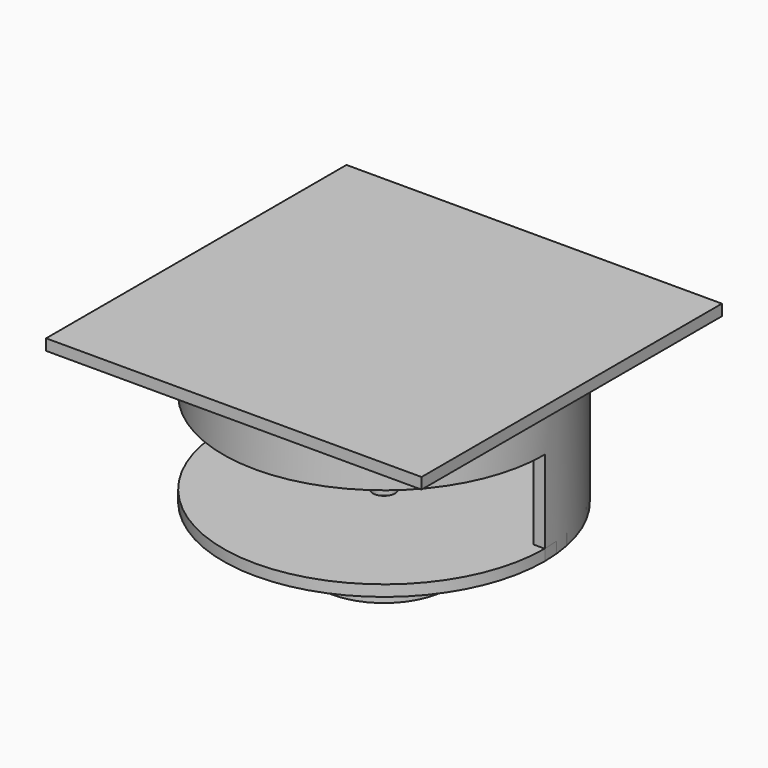
from build123d import *
from build123d import SkipClean  # not in build123d's __all__

# Parameters (mm, degrees)
F1_DEPTH  = 25.4
F2_DEPTH  = 3
F3_R      = 43.5
F3_R_2    = 40.5
F4_DEPTH  = 2
F5_R      = 43.5
F5_R_2    = 40.5
F6_DEPTH  = 12.7
F7_W      = 101.6
F7_H      = 101.6
F8_DEPTH  = 3
F9_R      = 17.5
F9_R_2    = 14
F10_DEPTH = 15
F11_D     = 6
F11_DEPTH = 20
F11_TIP   = 1.8025818571
F12_DEPTH = 3


# Not quite as in the source:
# - after a boolean that leaves OpenCascade's solid faulty, fix() repairs it
# - a feature names something its author has since deleted; it is built from what else it names


with BuildPart() as f1:
    # F0 (on Top) → F1 (new body)
    with BuildSketch(Plane.XY):
        with BuildLine():
            Line((0, 40.5), (0, 43.5))
            ThreePointArc((0, 43.5), (-30.7591449816, 30.7591449816), (-43.5, 0))
            Line((-43.5, 0), (-40.5, 0))
            ThreePointArc((-40.5, 0), (-28.6378246381, 28.6378246381), (0, 40.5))
        make_face()
        with BuildLine():
            Line((40.5, 0), (43.5, 0))
            ThreePointArc((43.5, 0), (30.7591449816, 30.7591449816), (0, 43.5))
            Line((0, 43.5), (0, 40.5))
            ThreePointArc((0, 40.5), (28.6378246381, 28.6378246381), (40.5, 0))
        make_face()
    extrude(amount=F1_DEPTH)

    # F3 (on face) → F4 (join)
    with BuildSketch(Plane.XY.offset(25.4)):
        Circle(F3_R)
        Circle(F3_R_2, mode=Mode.SUBTRACT)
    with SkipClean():  # cleaning this boolean's faces spoils the solid; the shape is the same uncleaned
        extrude(amount=F4_DEPTH)

    # F5 (on face) → F6 (join)
    with BuildSketch(Plane.XY.offset(27.4)):
        Circle(F5_R)
        Circle(F5_R_2, mode=Mode.SUBTRACT)
    extrude(amount=F6_DEPTH)

    add(f1.part.fix(), mode=Mode.REPLACE)

    # F7 (on face) → F8 (join)
    with BuildSketch(Plane.XY.offset(40.1)):
        Rectangle(F7_W, F7_H)
    extrude(amount=F8_DEPTH)


with BuildPart() as f2:
    # F0 (on Top) → F2 (new body)
    with BuildSketch(Plane.XY):
        with BuildLine():
            ThreePointArc((-43.5, 0), (0, -43.5), (43.5, 0))
            Line((43.5, 0), (40.5, 0))
            ThreePointArc((40.5, 0), (28.6378246381, 28.6378246381), (0, 40.5))
            ThreePointArc((0, 40.5), (-28.6378246381, 28.6378246381), (-40.5, 0))
            Line((-40.5, 0), (-43.5, 0))
        make_face()
    extrude(amount=F2_DEPTH)

    # F9 (on face) → F10 (join)
    with BuildSketch(Plane.XY):
        Circle(F9_R)
        Circle(F9_R_2, mode=Mode.SUBTRACT)
    extrude(amount=-F10_DEPTH)

    # F11
    with Locations(Plane(origin=(0, 0, 0), x_dir=(1, 0, 0), z_dir=(0, 0, -1))):
        with Locations((0, 0)):
            Hole(F11_D / 2, depth=F11_DEPTH)
            with Locations((0, 0, -(F11_DEPTH + F11_TIP / 2))):  # 118° drill point
                Cone(0, F11_D / 2, F11_TIP, mode=Mode.SUBTRACT)

    # F0 (on Top) → F12 (join)
    with BuildSketch(Plane.XY):
        with BuildLine():
            Line((0, 40.5), (0, 43.5))
            ThreePointArc((0, 43.5), (-30.7591449816, 30.7591449816), (-43.5, 0))
            Line((-43.5, 0), (-40.5, 0))
            ThreePointArc((-40.5, 0), (-28.6378246381, 28.6378246381), (0, 40.5))
        make_face()
        with BuildLine():
            Line((40.5, 0), (43.5, 0))
            ThreePointArc((43.5, 0), (30.7591449816, 30.7591449816), (0, 43.5))
            Line((0, 43.5), (0, 40.5))
            ThreePointArc((0, 40.5), (28.6378246381, 28.6378246381), (40.5, 0))
        make_face()
    extrude(amount=F12_DEPTH)


solid = Compound([f1.part, f2.part])
